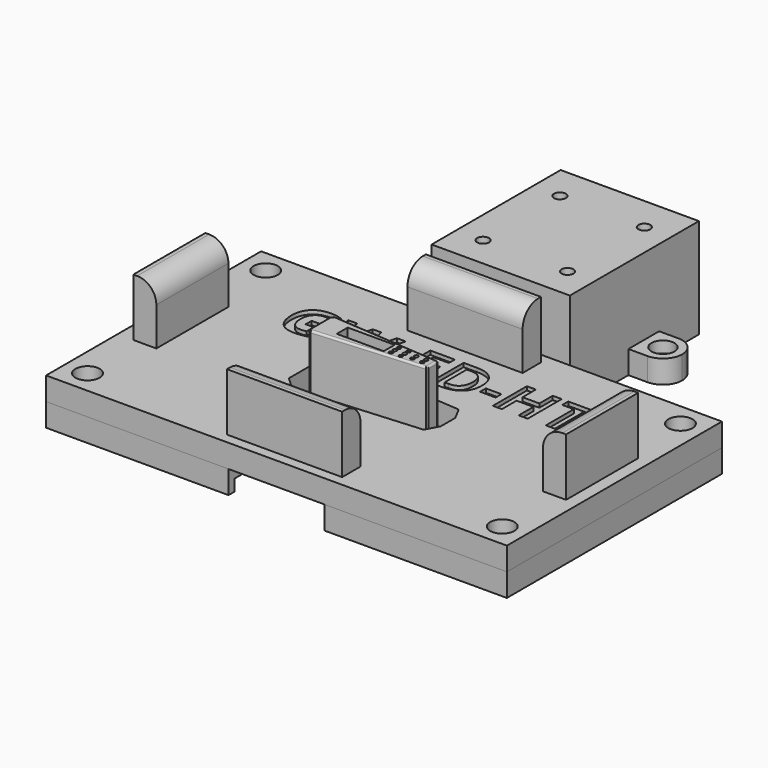
from build123d import *

# Parameters (mm, degrees)
F0_R          = 1.55
F0_W          = 10
F0_H          = 10
F1_DEPTH      = 6
F3_DEPTH      = 18
F4_R          = 0.5
F4_W          = 12.2195427539
F4_H          = 3.5648923367
F5_DEPTH      = 24.001
F7_DEPTH      = 10
F8_W          = 120
F8_H          = 70
F8_R          = 3.15
F9_DEPTH      = 6
F10_W         = 6
F10_H         = 23.4606322027
F10_W_2       = 30
F10_H_2       = 6
F11_DEPTH     = 15
F12_R         = 5
F13_R         = 0.5
F14_W         = 25
F14_H         = 5
F15_DEPTH     = 27.001
F16_W         = 62.6825769761
F16_H         = 31.7398100072
F17_DEPTH     = 3
F18_R         = 5.5
F19_DEPTH     = 2
F20_R         = 5.5
F21_DEPTH     = 2
F22_TEXT_SIZE = 15.5066944683
F23_DEPTH     = 1
F24_W         = 36
F24_H         = 42
F25_DEPTH     = 20
F26_R         = 1.55
F27_DEPTH     = 26.001
F28_R         = 3
F29_DEPTH     = 3
F30_R         = 4.99999


# Not quite as in the source:
# - a fillet or chamfer is up to 0.001 mm smaller than in the source, because OpenCascade refuses the exact size
# - Text() gives the source's letters only with a copy of the font that has no kerning and outlines rounded to 1/6400 em; it was checked with that copy


with BuildPart() as f1:
    # F0 (on Top) → F1 (new body)
    with BuildSketch(Plane.XY):
        Polygon((-18, 35), (-60, 35), (-60, -35), (60, -35), (60, 35), (18, 35), align=None)
        with Locations((-54, -29)):
            Circle(F0_R, mode=Mode.SUBTRACT)
        with Locations((-35, -28.9389491081)):
            Circle(F0_R, mode=Mode.SUBTRACT)
        with Locations((35, -28.9389491081)):
            Circle(F0_R, mode=Mode.SUBTRACT)
        with Locations((54, -29)):
            Circle(F0_R, mode=Mode.SUBTRACT)
        with Locations((-54, 29)):
            Circle(F0_R, mode=Mode.SUBTRACT)
        with Locations((54, 29)):
            Circle(F0_R, mode=Mode.SUBTRACT)
        Polygon((-18, 57.0610508919), (-18, 35), (18, 35), (18, 57.0610508919), (18, 67.0610508919), (18, 80), (-18, 80), (-18, 67.0610508919), align=None)
        with Locations((-23, 62.0610508919)):
            Rectangle(F0_W, F0_H)
        with Locations((-23, 62.0610508919)):
            Circle(F0_R, mode=Mode.SUBTRACT)
        with Locations((23, 62.0610508919)):
            Rectangle(F0_W, F0_H)
        with Locations((23, 62.0610508919)):
            Circle(F0_R, mode=Mode.SUBTRACT)
    extrude(amount=F1_DEPTH)

    # F2 (on face) → F3 (join)
    with BuildSketch(Plane.XY.offset(6)):
        Polygon((12.3937708153, -1.8799159334), (12.6722302646, -1.3554515159), (12.6722302646, 1.3554515159), (12.3937708153, 1.8799159334), (-15.9813273618, 4.0076783797), (-16.67, 3.3765164586), (-16.67, -3.3765164586), (-15.9813273618, -4.0076783797), align=None)
    extrude(amount=F3_DEPTH)

    # F4 (on face) → F5 (cut, through all)
    with BuildSketch(Plane.XY.offset(24)):
        with Locations((10.4722302646, 0.635)):
            Circle(F4_R)
        with Locations((10.4722302646, -0.635)):
            Circle(F4_R)
        with Locations((7.9322302646, 0.635)):
            Circle(F4_R)
        with Locations((7.9322302646, -0.635)):
            Circle(F4_R)
        with Locations((5.3922302646, 1.27)):
            Circle(F4_R)
        with Locations((5.3922302646, 0)):
            Circle(F4_R)
        with Locations((5.3922302646, -1.27)):
            Circle(F4_R)
        with Locations((2.8522302646, 1.27)):
            Circle(F4_R)
        with Locations((2.8522302646, 0)):
            Circle(F4_R)
        with Locations((2.8522302646, -1.27)):
            Circle(F4_R)
        with Locations((-4.7591286129, 0)):
            Rectangle(F4_W, F4_H)
    extrude(amount=-F5_DEPTH, mode=Mode.SUBTRACT)

    # F6 (on face) → F7 (cut)
    with BuildSketch(Plane(origin=(0, 0, 0), x_dir=(1, 0, 0), z_dir=(0, 0, -1))):
        Polygon((11.6383330896, 1.640868117), (0.7885956438, 2.3339718093), (0.7885956438, -2.3339718093), (11.6383330896, -1.640868117), align=None)
    extrude(amount=-F7_DEPTH, mode=Mode.SUBTRACT)

    # F13
    f13_edges = [f1.edges().sort_by_distance(p)[0] for p in [
        (-1.793778, -2.943797, 24),
        (-1.793778, 2.943797, 24),
        (12.67223, 0, 24),
        (12.533001, 1.617684, 24),
        (12.533001, -1.617684, 24),
        (-16.325664, -3.692097, 24),
        (-16.67, 0, 24),
        (-16.325664, 3.692097, 24),
    ]]
    fillet(f13_edges, radius=F13_R)

    # F14 (on face) → F15 (cut, through all)
    with BuildSketch(Plane(origin=(0, 0, 0), x_dir=(1, 0, 0), z_dir=(0, 0, -1))):
        with Locations((0, 32.5)):
            Rectangle(F14_W, F14_H)
    extrude(amount=-F15_DEPTH, mode=Mode.SUBTRACT)

    # F16 (on face) → F17 (cut)
    with BuildSketch(Plane(origin=(0, 0, 0), x_dir=(1, 0, 0), z_dir=(0, 0, -1))):
        with Locations((0, 17.1300949964)):
            Rectangle(F16_W, F16_H)
    extrude(amount=-F17_DEPTH, mode=Mode.SUBTRACT)

    # F18 (on face) → F19 (cut)
    with BuildSketch(Plane.XY.offset(6)):
        with Locations((-40, 20)):
            Circle(F18_R)
        with Locations((-40, -20)):
            Circle(F18_R)
        with Locations((40, -20)):
            Circle(F18_R)
        with Locations((40, 20)):
            Circle(F18_R)
    extrude(amount=-F19_DEPTH, mode=Mode.SUBTRACT)

    # F24 (on face) → F25 (join)
    with BuildSketch(Plane.XY.offset(6)):
        with Locations((0, 59)):
            Rectangle(F24_W, F24_H)
    extrude(amount=F25_DEPTH)

    # F26 (on face) → F27 (cut, through all)
    with BuildSketch(Plane.XY.offset(26)):
        with Locations((-11, 71)):
            Circle(F26_R)
        with Locations((11, 71)):
            Circle(F26_R)
        with Locations((-11, 46)):
            Circle(F26_R)
        with Locations((11, 46)):
            Circle(F26_R)
    extrude(amount=-F27_DEPTH, mode=Mode.SUBTRACT)

    # F28 (on face) → F29 (cut)
    with BuildSketch(Plane.XY.offset(6)):
        with Locations((-35, -28.9389491081)):
            Circle(F28_R)
        with Locations((35, -28.9389491081)):
            Circle(F28_R)
        with Locations((23, 62.0610508919)):
            Circle(F28_R)
        with Locations((-23, 62.0610508919)):
            Circle(F28_R)
    extrude(amount=-F29_DEPTH, mode=Mode.SUBTRACT)

    # F30 (radius 5 in the source; OpenCascade refuses exactly that, so slightly less here)
    f30_edges = [f1.edges().sort_by_distance(p)[0] for p in [
        (-28, 57.061051, 3),
        (-28, 67.061051, 3),
        (28, 57.061051, 3),
        (28, 67.061051, 3),
    ]]
    fillet(f30_edges, radius=F30_R)


with BuildPart() as f9:
    # F8 (on face) → F9 (new body)
    with BuildSketch(Plane.XY.offset(6)):
        Rectangle(F8_W, F8_H)
        with Locations((-54, -29)):
            Circle(F8_R, mode=Mode.SUBTRACT)
        with Locations((54, -29)):
            Circle(F8_R, mode=Mode.SUBTRACT)
        Polygon((-17.4080537441, -8.1258945829), (-20.67, -5.1363518727), (-20.67, 5.1363518727), (-17.4080537441, 8.1258945829), (14.8923609567, 5.7037845704), (16.6722302646, 2.3514899299), (16.6722302646, -2.3514899299), (14.8923609567, -5.7037845704), align=None, mode=Mode.SUBTRACT)
        with Locations((-54, 29)):
            Circle(F8_R, mode=Mode.SUBTRACT)
        with Locations((54, 29)):
            Circle(F8_R, mode=Mode.SUBTRACT)
    extrude(amount=F9_DEPTH)

    # F10 (on face) → F11 (join)
    with BuildSketch(Plane.XY.offset(12)):
        with Locations((-52.9, 0)):
            Rectangle(F10_W, F10_H)
        with Locations((0, 29.375)):
            Rectangle(F10_W_2, F10_H_2)
        with Locations((0, -29.375)):
            Rectangle(F10_W_2, F10_H_2)
        with Locations((53.8, 0)):
            Rectangle(F10_W, F10_H)
    extrude(amount=F11_DEPTH)

    # F12
    f12_edges = [f9.edges().sort_by_distance(p)[0] for p in [
        (0, -26.375, 27),
        (-49.9, 0, 27),
        (0, 26.375, 27),
        (50.8, 0, 27),
    ]]
    fillet(f12_edges, radius=F12_R)

    # F20 (on face) → F21 (cut)
    with BuildSketch(Plane(origin=(0, 0, 6), x_dir=(1, 0, 0), z_dir=(0, 0, -1))):
        with Locations((-40, 20)):
            Circle(F20_R)
        with Locations((-40, -20)):
            Circle(F20_R)
        with Locations((40, -20)):
            Circle(F20_R)
        with Locations((40, 20)):
            Circle(F20_R)
    extrude(amount=-F21_DEPTH, mode=Mode.SUBTRACT)

    # F22 (on face) → F23 (cut)
    with BuildSketch(Plane.XY.offset(12)):
        with Locations((-38.4481220578, 11.3012378944)):
            Text('GW-ED-HT', F22_TEXT_SIZE, font='Open Sans', font_style=FontStyle.BOLD, text_align=(TextAlign.LEFT, TextAlign.BOTTOM))
    extrude(amount=-F23_DEPTH, mode=Mode.SUBTRACT)


with BuildPart() as f31_1:
    # F31: copy of F1
    add(f1.part)


solid = Compound([f1.part, f9.part])
